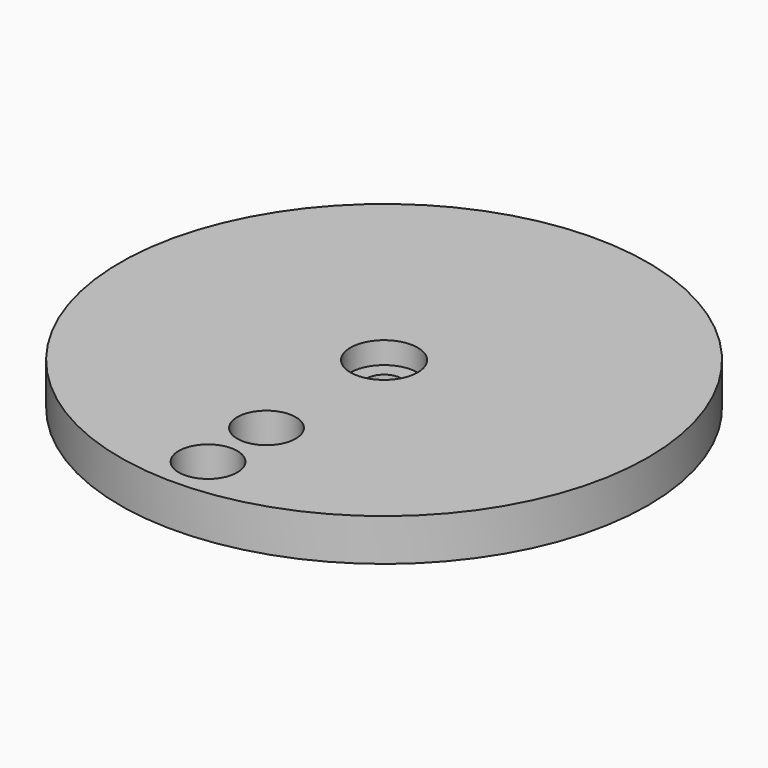
from build123d import *

# Parameters (mm, degrees)
F0_R     = 22.9235
F1_DEPTH = 3.6576
F2_R     = 2.54
F3_DEPTH = 3.6586
F2_R_2   = 1.524
F4_DEPTH = 25.4
F5_R     = 2.921
F5_R_2   = 1.524
F6_DEPTH = 1.905


# Not quite as in the source:
# - a feature names something its author has since deleted; it is built from what else it names


with BuildPart() as f1:
    # F0 (on Top) → F1 (new body)
    with BuildSketch(Plane.XY):
        Circle(F0_R)
    extrude(amount=F1_DEPTH)

    # F2 (on face) → F3 (cut, through all)
    with BuildSketch(Plane.XY.offset(3.6576)):
        with Locations((0, -19.1135)):
            Circle(F2_R)
        with Locations((0, -12.7635)):
            Circle(F2_R)
    extrude(amount=-F3_DEPTH, mode=Mode.SUBTRACT)

    # F2 (on face) → F4 (cut)
    with BuildSketch(Plane.XY.offset(3.6576)):
        Circle(F2_R_2)
    extrude(amount=-F4_DEPTH, mode=Mode.SUBTRACT)

    # F5 (on face) → F6 (cut)
    with BuildSketch(Plane.XY.offset(3.6576)):
        Circle(F5_R)
        Circle(F5_R_2, mode=Mode.SUBTRACT)
    extrude(amount=-F6_DEPTH, mode=Mode.SUBTRACT)


solid = f1.part
